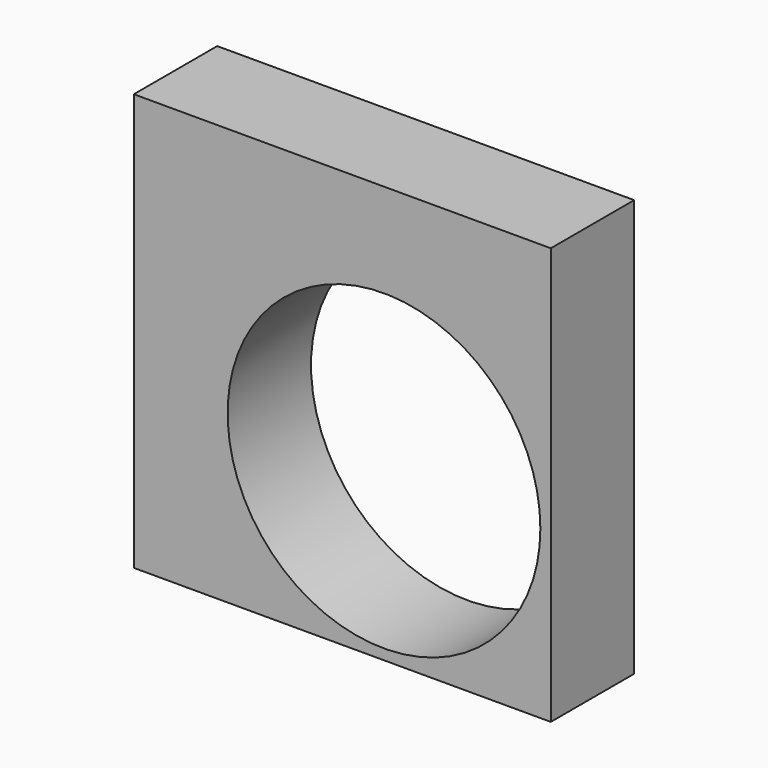
from build123d import *

# Parameters (mm, degrees)
F0_W     = 101.6
F0_H     = 101.6
F1_DEPTH = 25.4
F2_R     = 38.1
F3_DEPTH = 25.4


# Not quite as in the source:
# - a feature names something its author has since deleted; it is built from what else it names


with BuildPart() as f1:
    # F0 (on Front) → F1 (new body)
    with BuildSketch(Plane.XZ):
        Rectangle(F0_W, F0_H)
    extrude(amount=F1_DEPTH)

    # F2 (on face) → F3 (cut)
    with BuildSketch(Plane.XZ.offset(25.4)):
        with Locations((10.16, -10.16)):
            Circle(F2_R)
    extrude(amount=-F3_DEPTH, mode=Mode.SUBTRACT)


solid = f1.part
